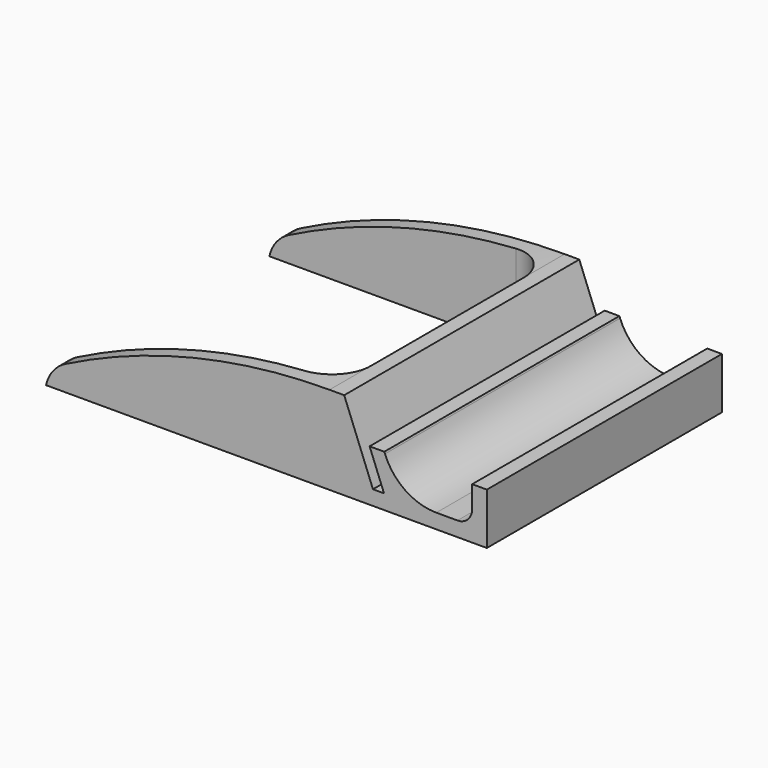
from build123d import *

# Parameters (mm, degrees)
F1_DEPTH    = 40
F2_R        = 7.5
F3_R        = 2
F4_W        = 38.5823002379
F4_H        = 36
F5_DEPTH    = 25.4
F6_R        = 5
F7_T1_DEPTH = 16.8444406885
F7_T3_DEPTH = 16.8444406885


# Not quite as in the source:
# - a fillet or chamfer that OpenCascade refuses, or shapes differently, is made with other operations: its cross-section is extruded or revolved along the edge and cut away or added


with BuildPart() as f1:
    # F0 (on Front) → F1 (new body)
    with BuildSketch(Plane.XZ):
        with BuildLine():
            ThreePointArc((-19.4176997621, 10), (-39.3462840799, 7.4593677642), (-58, 0))
            Line((-58, 0), (-19.4176997621, 0))
            Line((-19.4176997621, 0), (-19.4176997621, 10))
        make_face()
        Polygon((0, 5), (0, 0), (-10, 0), (-11.9571349147, 5), (-13.9571349147, 5), (-12, 0), (-13.5034299327, 0), (-17.4176997621, 10), (-19.4176997621, 10), (-19.4176997621, 0), (-58, 0), (-58, -2), (2, -2), (2, 5), align=None)
    extrude(amount=-F1_DEPTH)

    # F2
    f2_edges = [f1.edges().sort_by_distance(p)[0] for p in [
        (-10, 20, 0),
    ]]
    fillet(f2_edges, radius=F2_R)

    # F3
    f3_edges = [f1.edges().sort_by_distance(p)[0] for p in [
        (0, 20, 0),
    ]]
    fillet(f3_edges, radius=F3_R)

    # F4 (on face) → F5 (cut)
    with BuildSketch(Plane.XY.offset(10)):
        with Locations((-38.7088498811, 20)):
            Rectangle(F4_W, F4_H)
    extrude(amount=-F5_DEPTH, mode=Mode.SUBTRACT)

    # F6
    f6_edges = [f1.edges().sort_by_distance(p)[0] for p in [
        (-19.4177, 2, 4),
        (-19.4177, 38, 4),
    ]]
    fillet(f6_edges, radius=F6_R)

    # F7: fillet of radius 5 on 2 edges, made by hand

    # F7_s2 → F7_t1 (cut)
    with BuildSketch(Plane.XZ.offset(-9.4222203443)):
        with BuildLine():
            ThreePointArc((-58, -2), (-57.0714339554, -0.0080127697), (-55.3783893775, 1.3933608716))
            ThreePointArc((-55.3783893775, 1.3933608716), (-56.6957053109, 0.7089301814), (-58, 0))
            Line((-58, 0), (-58, -2))
        make_face()
    extrude(amount=F7_T1_DEPTH, mode=Mode.SUBTRACT)

    # F7_s4 → F7_t3 (cut)
    with BuildSketch(Plane.XZ.offset(-47.4222203443)):
        with BuildLine():
            ThreePointArc((-58, -2), (-57.0714339554, -0.0080127697), (-55.3783893775, 1.3933608716))
            ThreePointArc((-55.3783893775, 1.3933608716), (-56.6957053109, 0.7089301814), (-58, 0))
            Line((-58, 0), (-58, -2))
        make_face()
    extrude(amount=F7_T3_DEPTH, mode=Mode.SUBTRACT)


solid = f1.part
